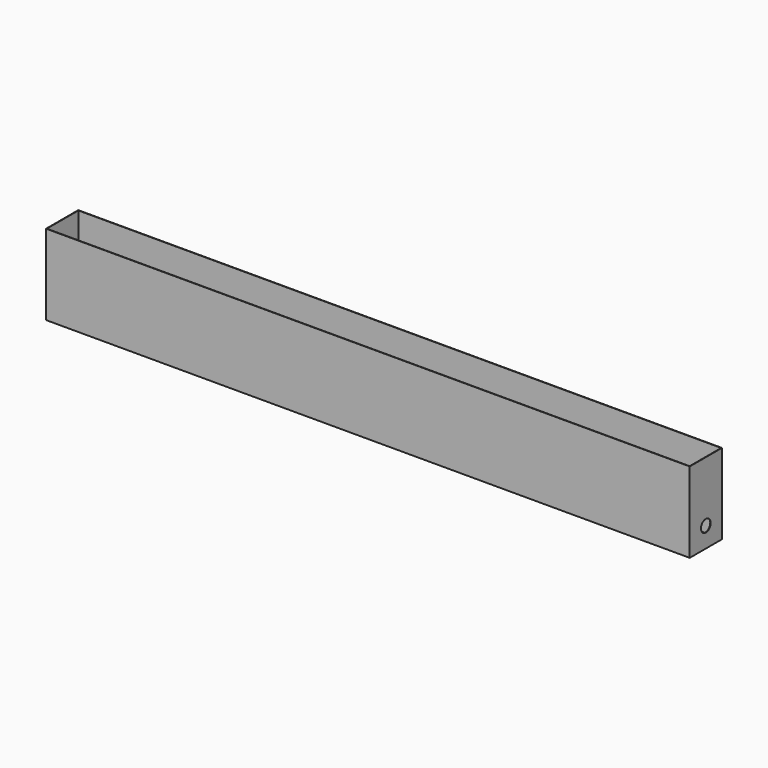
from build123d import *

# Parameters (mm, degrees)
F0_W     = 1600
F0_H     = 100
F1_DEPTH = 200
F2_T     = -1
F5_D     = 20
F8_D     = 30


# Not quite as in the source:
# - the program builds the solid bodies; features that only make, move or delete a surface that nothing else refers to are left out


with BuildPart() as f1:
    # F0 (on Top) → F1 (new body)
    with BuildSketch(Plane.XY):
        Rectangle(F0_W, F0_H)
    extrude(amount=F1_DEPTH)

    # F2
    f2_openings = [f1.faces().sort_by_distance(p)[0] for p in [
        (0, 0, 200),
    ]]
    offset(amount=F2_T, openings=f2_openings)

    # F5 (through all)
    with Locations(Plane.XY.offset(1)):
        with Locations((787, 37), (787, -37), (-787, 37), (-787, -37)):
            Hole(F5_D / 2)

    # F8 (through all)
    with Locations(Plane(origin=(-800, 0, 0), x_dir=(0, -1, 0), z_dir=(-1, 0, 0))):
        with Locations((0, 50)):
            Hole(F8_D / 2)


solid = f1.part
